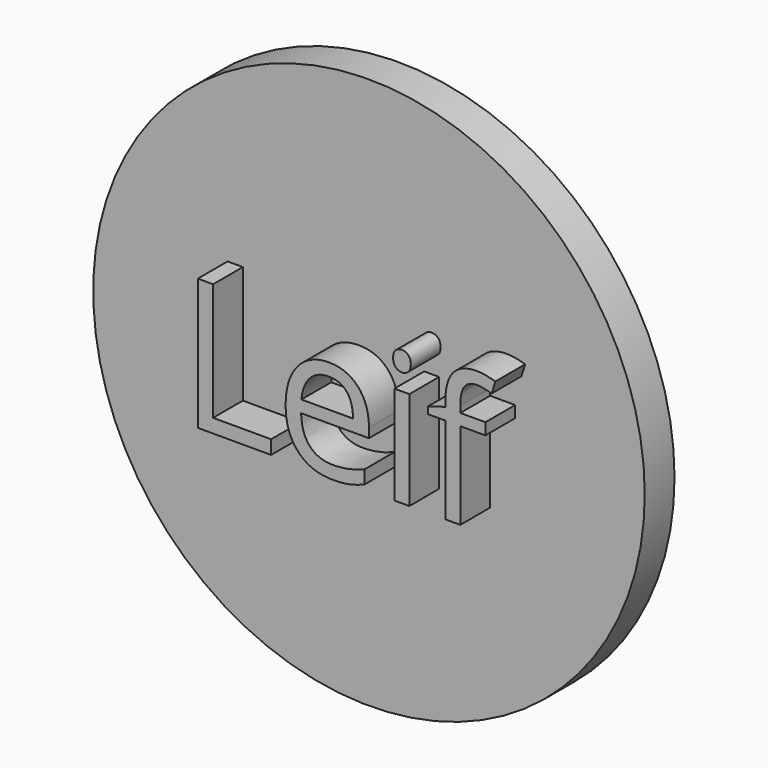
from build123d import *

# Parameters (mm, degrees)
F0_R         = 74.0608739771
F1_DEPTH     = 10
F2_TEXT_SIZE = 49.4368555438
F3_DEPTH     = 10


# Not quite as in the source:
# - Text() gives the source's letters only with a copy of the font that has no kerning and outlines rounded to 1/6400 em; it was checked with that copy


with BuildPart() as f1:
    # F0 (on Front) → F1 (new body)
    with BuildSketch(Plane.XZ):
        Circle(F0_R)
    extrude(amount=F1_DEPTH)

    # F2 (on face) → F3 (join)
    with BuildSketch(Plane.XZ.offset(10)):
        with Locations((-42.8163377801, -16.6340470314)):
            Text('Leif', F2_TEXT_SIZE, font='Open Sans', text_align=(TextAlign.LEFT, TextAlign.BOTTOM))
    extrude(amount=F3_DEPTH)


solid = f1.part
